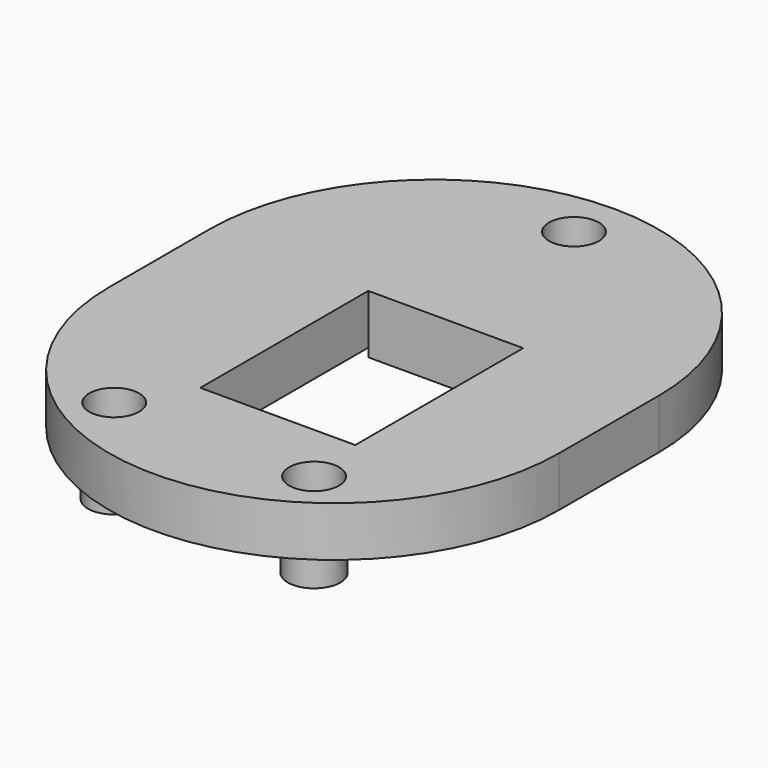
from build123d import *

# Parameters (mm, degrees)
F1_DEPTH    = 10
F3_R        = 44.99999
F4_W        = 31
F4_H        = 42
F5_DEPTH    = 11
F6_R        = 5.25
F7_DEPTH    = 7
F9_D        = 10
F9_DEPTH    = 10.001
F10_D       = 6.5
F10_ON_F6_D = 6.5
F11_W       = 31
F11_H       = 2.5
F12_DEPTH   = 1.7


# Not quite as in the source:
# - a fillet or chamfer is up to 0.001 mm smaller than in the source, because OpenCascade refuses the exact size


with BuildPart() as f1:
    # F0 (on Top) → F1 (new body)
    with BuildSketch(Plane.XY):
        with BuildLine():
            Line((-45, 70), (-45, 0))
            ThreePointArc((-45, 0), (0, -45), (45, 0))
            Line((45, 0), (45, 70))
            Line((45, 70), (-45, 70))
        make_face()
    extrude(amount=F1_DEPTH)

    # F3 (radius 45 in the source; OpenCascade refuses exactly that, so slightly less here)
    f3_edges = [f1.edges().sort_by_distance(p)[0] for p in [
        (-45, 70, 5),
        (45, 70, 5),
    ]]
    fillet(f3_edges, radius=F3_R)

    # F4 (on face) → F5 (cut)
    with BuildSketch(Plane.XY.offset(10)):
        with Locations((2.9, 3.3)):
            Rectangle(F4_W, F4_H)
    extrude(amount=-F5_DEPTH, mode=Mode.SUBTRACT)

    # F6 (on face) → F7 (join)
    with BuildSketch(Plane(origin=(0, 0, 0), x_dir=(1, 0, 0), z_dir=(0, 0, -1))):
        with Locations((0, -60)):
            Circle(F6_R)
        with Locations((-20, 30)):
            Circle(F6_R)
        with Locations((20, 30)):
            Circle(F6_R)
    extrude(amount=F7_DEPTH)

    # F9 (through all, one way)
    with BuildSketch(Plane(origin=(0, 0, 0), x_dir=(1, 0, 0), z_dir=(0, 0, -1))):
        with Locations((-20, 30), (20, 30), (0, -60)):
            Circle(F9_D / 2)
    extrude(amount=-F9_DEPTH, mode=Mode.SUBTRACT)

    # F10 (through all)
    with Locations(Plane.XY):
        with Locations((20, -30), (0, 60)):
            Hole(F10_D / 2)

    # F10 on F6 (through all)
    with Locations(Plane.XY):
        with Locations((-20, -30)):
            Hole(F10_ON_F6_D / 2)

    # F11 (on face) → F12 (join)
    with BuildSketch(Plane(origin=(0, 0, 0), x_dir=(1, 0, 0), z_dir=(0, 0, -1))):
        with Locations((2.9, -25.55)):
            Rectangle(F11_W, F11_H)
    extrude(amount=F12_DEPTH)


solid = f1.part
